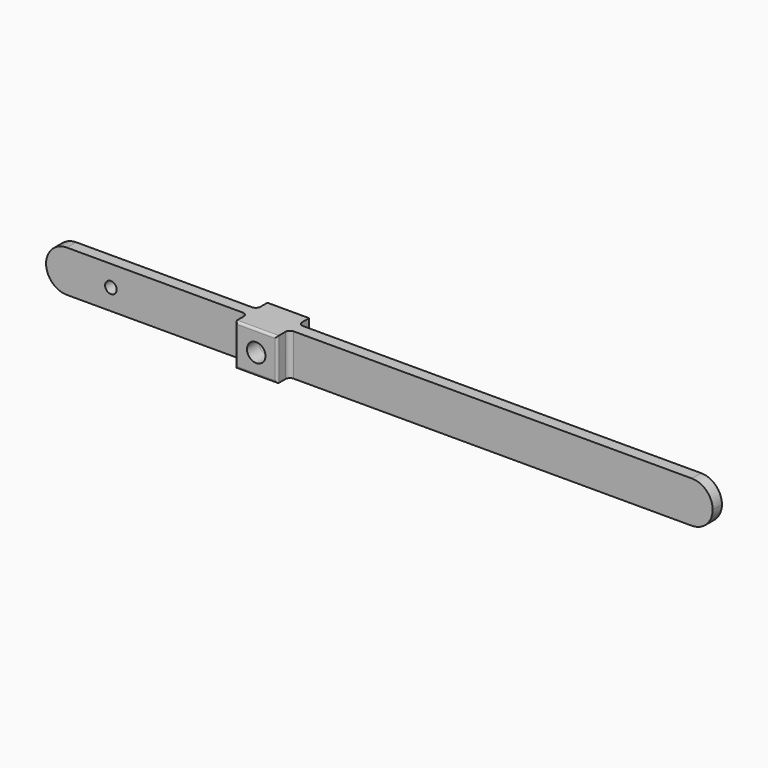
from build123d import *

# Parameters (mm, degrees)
F1_DEPTH = 57.15
F2_R     = 3.175
F3_R     = 28.57499
F4_R     = 28.575
F5_R     = 28.57499
F7_D     = 15.875
F8_D     = 25.4
F8_DEPTH = 38.1
F8_TIP   = 7.6309298617
F9_D     = 25.4


# Not quite as in the source:
# - a fillet or chamfer is up to 0.001 mm smaller than in the source, because OpenCascade refuses the exact size
# - a length typed as a fraction of an inch, garbled in the dataset ("3 / 203.2 mm" for 3/8 in), is restored


with BuildPart() as f1:
    # F0 (on Top) → F1 (new body)
    with BuildSketch(Plane.XY):
        with BuildLine():
            ThreePointArc((28.575, -6.35), (30.4348719395, -1.8598719395), (34.925, 0))
            Line((34.925, 0), (609.6, 0))
            Line((609.6, 0), (609.6, 15.875))
            Line((609.6, 15.875), (34.925, 15.875))
            ThreePointArc((34.925, 15.875), (30.4348719395, 17.7348719395), (28.575, 22.225))
            Line((28.575, 22.225), (28.575, 36.5125))
            Line((28.575, 36.5125), (0, 36.5125))
            Line((0, 36.5125), (-28.575, 36.5125))
            Line((-28.575, 36.5125), (-28.575, 22.225))
            ThreePointArc((-28.575, 22.225), (-30.4348719395, 17.7348719395), (-34.925, 15.875))
            Line((-34.925, 15.875), (-304.8, 15.875))
            Line((-304.8, 15.875), (-304.8, 0))
            Line((-304.8, 0), (-34.925, 0))
            ThreePointArc((-34.925, 0), (-30.4348719395, -1.8598719395), (-28.575, -6.35))
            Line((-28.575, -6.35), (-28.575, -20.6375))
            Line((-28.575, -20.6375), (0, -20.6375))
            Line((0, -20.6375), (28.575, -20.6375))
            Line((28.575, -20.6375), (28.575, -6.35))
        make_face()
    extrude(amount=F1_DEPTH)

    # F2
    f2_edges = [f1.edges().sort_by_distance(p)[0] for p in [
        (28.575, 36.5125, 28.575),
        (0, 36.5125, 57.15),
        (-28.575, 36.5125, 28.575),
        (0, 36.5125, 0),
        (-28.575, -20.6375, 28.575),
        (0, -20.6375, 57.15),
        (28.575, -20.6375, 28.575),
        (0, -20.6375, 0),
    ]]
    fillet(f2_edges, radius=F2_R)

    # F3 (radius 28.575 in the source; OpenCascade refuses exactly that, so slightly less here)
    f3_edges = [f1.edges().sort_by_distance(p)[0] for p in [
        (-304.8, 7.9375, 57.15),
        (-304.8, 7.9375, 0),
    ]]
    fillet(f3_edges, radius=F3_R)

    # F4
    f4_edges = [f1.edges().sort_by_distance(p)[0] for p in [
        (609.6, 7.9375, 57.15),
    ]]
    fillet(f4_edges, radius=F4_R)

    # F5 (radius 28.575 in the source; OpenCascade refuses exactly that, so slightly less here)
    f5_edges = [f1.edges().sort_by_distance(p)[0] for p in [
        (609.6, 7.9375, 0),
    ]]
    fillet(f5_edges, radius=F5_R)

    # F7 (through all)
    with Locations(Plane.XZ):
        with Locations((-215.9, 28.575)):
            Hole(F7_D / 2)

    # F8 (one way)
    with BuildSketch(Plane.XZ):
        with Locations((0, 28.575)):
            Circle(F8_D / 2)
    extrude(amount=-F8_DEPTH, mode=Mode.SUBTRACT)
    with Locations(Plane.XZ):
        with Locations((0, 28.575)):
            with Locations((0, 0, -(F8_DEPTH + F8_TIP / 2))):  # 118° drill point
                Cone(0, F8_D / 2, F8_TIP, mode=Mode.SUBTRACT)

    # F9 (through all)
    with Locations(Plane(origin=(0, 0, 0), x_dir=(1, 0, 0), z_dir=(0, 1, 0))):
        with Locations((0, -28.575)):
            Hole(F9_D / 2)


solid = f1.part
